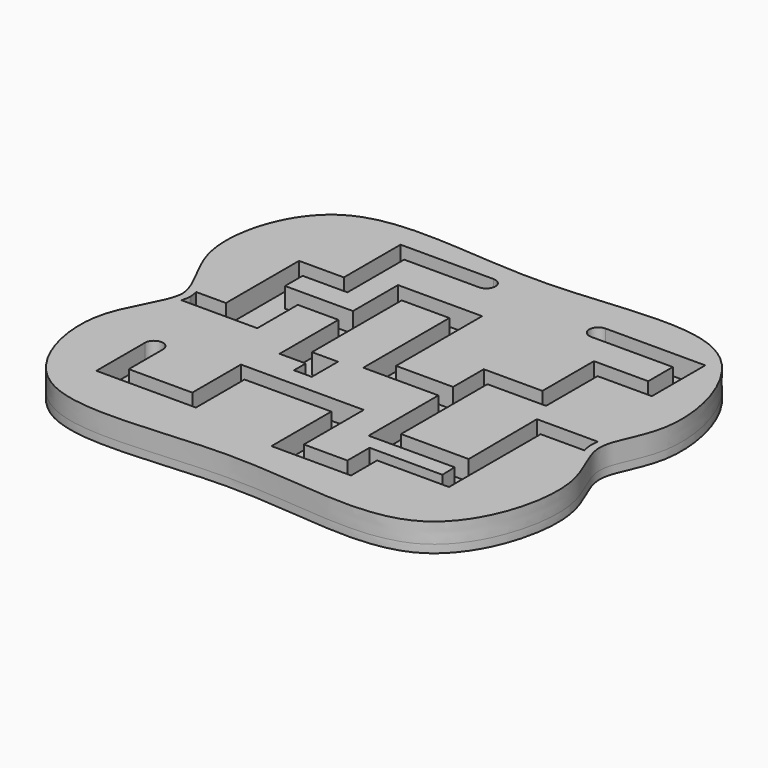
from build123d import *

# Parameters (mm, degrees)
F1_DEPTH = 5
F3_DEPTH = 2


# Not quite as in the source:
# - ends of sketch curves that miss each other by under 0.0002 mm in the source are joined
# - the dataset's text gives a spline's control points without its knots; the knots are read off the source's solid


with BuildPart() as f1:
    # F0 (on Top) → F1 (new body)
    with BuildSketch(Plane.XY):
        with BuildLine():
            add(Edge.make_bspline(
                [(-50.9456880391, 0), (-51.503372077, 5.566100958), (-62.5146563062, 16.7687371178), (-51.6356678734, 55.8412478467), (0.1475571881, 42.8791360776), (50.2128520626, 56.7362917081), (62.2679110659, 14.7606837887), (53.2085513997, 4.423548849), (53.2085513997, 0)],
                knots=[0, 0, 0, 0, 0.1323057261, 0.2944464696, 0.5028679611, 0.7079205641, 0.8788275568, 1, 1, 1, 1], degree=3))
            add(Edge.make_bspline(
                [(-50.9456880391, 0), (-51.503372077, -5.566100958), (-62.5146563062, -16.7687371178), (-51.6356678734, -55.8412478467), (0.1475571881, -42.8791360776), (50.2128520626, -56.7362917081), (62.2679110659, -14.7606837887), (53.2085513997, -4.423548849), (53.2085513997, 0)],
                knots=[0, 0, 0, 0, 0.1323057261, 0.2944464696, 0.5028679611, 0.7079205641, 0.8788275568, 1, 1, 1, 1], degree=3))
        make_face()
        with BuildLine():
            Line((-48.9556517112, -0.199387597), (-48.9556517112, 0.199387597))
            add(Edge.make_bspline(
                [(-48.9556517112, 0.199387597), (-49.0230581408, 0.872153835), (-49.1434598402, 1.5283549669), (-49.3032455355, 2.1689208225)],
                knots=[0, 0, 0, 0, 0.0134565679, 0.0134565679, 0.0134565679, 0.0134565679], degree=3))
            add(Edge.make_bspline(
                [(-49.3032455355, 2.1689208225), (-49.3289938856, 2.2721435415), (-49.5486681117, 3.1158233145), (-50.3333765859, 5.3666022776), (-51.7083191736, 8.0724029733), (-53.1209086073, 10.7900166471), (-54.129106738, 12.8665682522), (-55.0170217752, 15.0110037787), (-55.6046051051, 16.8816712621), (-55.9522945748, 18.4420782969), (-56.2119350784, 20.0683796187), (-56.3724776346, 22.2239468518), (-56.2956181819, 24.9357462684), (-55.9484823091, 27.7099356689), (-55.3327645413, 30.4826837202), (-54.1596605839, 34.0951290577), (-52.4706173692, 37.4569548645), (-50.3055678721, 40.3373443598), (-48.7651043366, 41.8945148544), (-47.4239283107, 42.9732523053), (-46.3668717243, 43.6917267161), (-45.2431785, 44.3276277734), (-42.8583955664, 45.4469740118), (-38.7592709718, 46.5788205426), (-32.3058608948, 47.1262089229), (-25.0820855304, 46.9759496812), (-17.2930636884, 46.4412854792), (-10.4881214189, 45.9507506166), (-4.9427269682, 45.7017808464), (-1.4517359227, 45.6414313985), (1.3455768971, 45.6739189351), (4.1268429052, 45.7580649245), (7.5730162875, 45.9432190449), (11.6414290853, 46.2478539423), (16.9540360773, 46.7029916702), (23.3402489636, 47.2508675251), (30.4419879804, 47.5223937353), (36.811225819, 47.0752312205), (41.3600698997, 45.8689935004), (44.1162047486, 44.4839190145), (45.5724511014, 43.5193095702), (46.9701029127, 42.4225154001), (48.6041529452, 40.8189337724), (50.9584744577, 37.8205240312), (53.3730883469, 33.4014157471), (55.3284302579, 27.5244590296), (56.1242091362, 22.5860447114), (56.2480403548, 18.8831588665), (56.1134124796, 16.729489546), (55.8816325113, 15.1445697663), (55.5699441853, 13.625327009), (55.0539456622, 11.8342505962), (54.297765853, 9.8121817564), (53.4729568569, 7.8763608061), (52.6525822662, 5.983449899), (51.9178222861, 4.0821512315), (51.5184265331, 2.6556326514), (51.3750938957, 1.8579303284), (51.35575883, 1.7403489352)],
                knots=[0.0134565679, 0.0134565679, 0.0134565679, 0.0134565679, 0.015625, 0.03125, 0.0625, 0.078125, 0.09375, 0.109375, 0.125, 0.1328125, 0.140625, 0.15625, 0.171875, 0.1875, 0.203125, 0.21875, 0.25, 0.265625, 0.28125, 0.2890625, 0.296875, 0.3046875, 0.3125, 0.34375, 0.375, 0.40625, 0.4375, 0.46875, 0.484375, 0.5, 0.5078125, 0.515625, 0.53125, 0.546875, 0.5625, 0.59375, 0.625, 0.65625, 0.6875, 0.703125, 0.7109375, 0.71875, 0.734375, 0.75, 0.78125, 0.8125, 0.84375, 0.859375, 0.875, 0.8828125, 0.890625, 0.90625, 0.921875, 0.9375, 0.953125, 0.96875, 0.984375, 0.9870602893, 0.9870602893, 0.9870602893, 0.9870602893], degree=3))
            add(Edge.make_bspline(
                [(51.35575883, 1.7403489352), (51.2698747401, 1.2180662045), (51.2172428231, 0.684051253), (51.2095357831, 0.1389744246)],
                knots=[0.9870602893, 0.9870602893, 0.9870602893, 0.9870602893, 0.9989880287, 0.9989880287, 0.9989880287, 0.9989880287], degree=3))
            Line((51.2095357831, 0.1389744246), (51.2085513997, 0))
            add(Edge.make_bspline(
                [(51.5661417074, -2.7596510648), (51.511731272, -2.5389008313), (51.3135124198, -1.6457876627), (51.2085513997, -0.7164876933), (51.2085513997, 0)],
                knots=[0.9791854168, 0.9791854168, 0.9791854168, 0.9791854168, 0.984375, 1, 1, 1, 1], degree=3))
            add(Edge.make_bspline(
                [(-49.3446149503, -2.3310785091), (-49.3573549812, -2.3799350681), (-49.566873924, -3.1680430377), (-50.3333765859, -5.3666022776), (-51.7083191736, -8.0724029733), (-53.1209086073, -10.7900166471), (-54.129106738, -12.8665682522), (-55.0170217752, -15.0110037787), (-55.6046051051, -16.8816712621), (-55.9522945748, -18.4420782969), (-56.2119350784, -20.0683796187), (-56.3724776346, -22.2239468518), (-56.2956181819, -24.9357462684), (-55.9484823091, -27.7099356689), (-55.3327645413, -30.4826837202), (-54.1596605839, -34.0951290577), (-52.4706173692, -37.4569548645), (-50.3055678721, -40.3373443598), (-48.7651043366, -41.8945148544), (-47.4239283107, -42.9732523053), (-46.3668717243, -43.6917267161), (-45.2431785, -44.3276277734), (-42.8583955664, -45.4469740118), (-38.7592709718, -46.5788205426), (-32.3058608948, -47.1262089229), (-25.0820855304, -46.9759496812), (-17.2930636884, -46.4412854792), (-10.4881214189, -45.9507506166), (-4.9427269682, -45.7017808464), (-1.4517359227, -45.6414313985), (1.3455768971, -45.6739189351), (4.1268429052, -45.7580649245), (7.5730162875, -45.9432190449), (11.6414290853, -46.2478539423), (16.9540360773, -46.7029916702), (23.3402489636, -47.2508675251), (30.4419879804, -47.5223937353), (36.811225819, -47.0752312205), (41.3600698997, -45.8689935004), (44.1162047486, -44.4839190145), (45.5724511014, -43.5193095702), (46.9701029127, -42.4225154001), (48.6041529452, -40.8189337724), (50.9584744577, -37.8205240312), (53.3730883469, -33.4014157471), (55.3284302579, -27.5244590296), (56.1242091362, -22.5860447114), (56.2480403548, -18.8831588665), (56.1134124796, -16.729489546), (55.8816325113, -15.1445697663), (55.5699441853, -13.625327009), (55.0539456622, -11.8342505962), (54.297765853, -9.8121817564), (53.4729568569, -7.8763608061), (52.6525822662, -5.983449899), (51.9991683774, -4.292646113), (51.6755523391, -3.2035442686), (51.5661417074, -2.7596510648)],
                knots=[0.0145944116, 0.0145944116, 0.0145944116, 0.0145944116, 0.015625, 0.03125, 0.0625, 0.078125, 0.09375, 0.109375, 0.125, 0.1328125, 0.140625, 0.15625, 0.171875, 0.1875, 0.203125, 0.21875, 0.25, 0.265625, 0.28125, 0.2890625, 0.296875, 0.3046875, 0.3125, 0.34375, 0.375, 0.40625, 0.4375, 0.46875, 0.484375, 0.5, 0.5078125, 0.515625, 0.53125, 0.546875, 0.5625, 0.59375, 0.625, 0.65625, 0.6875, 0.703125, 0.7109375, 0.71875, 0.734375, 0.75, 0.78125, 0.8125, 0.84375, 0.859375, 0.875, 0.8828125, 0.890625, 0.90625, 0.921875, 0.9375, 0.953125, 0.96875, 0.9791854168, 0.9791854168, 0.9791854168, 0.9791854168], degree=3))
            add(Edge.make_bspline(
                [(-48.9556517112, -0.199387597), (-49.0287578091, -0.9290407592), (-49.1642003, -1.6392089944), (-49.3446149503, -2.3310785091)],
                knots=[0, 0, 0, 0, 0.0145944116, 0.0145944116, 0.0145944116, 0.0145944116], degree=3))
        make_face(mode=Mode.SUBTRACT)
        with BuildLine():
            Line((-13.7496860698, -11.7393117398), (-13.7558765718, -11.7393396612))
            Line((-13.7558765718, -11.7393396612), (-23.7765221646, -11.784536536))
            Line((-23.7765221646, -11.784536536), (-23.7765440643, -4.1925245896))
            Line((-23.7765440643, -4.1925245896), (-45.4828031361, -4.1925245896))
            ThreePointArc((-45.4828031361, -4.1925245896), (-47.7328031361, -6.4425245896), (-45.4828031361, -8.6925245896))
            Line((-45.4828031361, -8.6925245896), (-28.2765440643, -8.6925245896))
            Line((-28.2765440643, -8.6925245896), (-28.2765440643, -16.3048788162))
            Line((-28.2765440643, -16.3048788162), (-23.3427176327, -16.2988154143))
            Line((-23.3427176327, -16.2988154143), (7.32941553, -16.2988154143))
            Line((7.32941553, -16.2988154143), (7.32941553, -34.9776947796))
            Line((7.32941553, -34.9776947796), (18.1962005645, -34.9776947796))
            Line((18.1962005645, -34.9776947796), (18.1962005645, -28.0615705997))
            Line((18.1962005645, -28.0615705997), (36.4300050671, -28.1137742644))
            Line((36.4300050671, -28.1137742644), (36.3082401454, -24.1376161575))
            Line((36.3082401454, -24.1376161575), (14.8714620192, -24.2085577739))
            Line((14.8714620192, -24.2085577739), (14.8714620192, -2.4310778646))
            Line((14.8714620192, -2.4310778646), (-3.8760740971, -2.4310778646))
            Line((-3.8760740971, -2.4310778646), (-3.8760740971, 24.4457749831))
            Line((-3.8760740971, 24.4457749831), (-15.7917661872, 24.4457749831))
            Line((-15.7917661872, 24.4457749831), (-15.7917661872, 10.4851193981))
            Line((-15.7917661872, 10.4851193981), (-15.7917661872, -3.5465050414))
            Line((-15.7917661872, -3.5465050414), (-9.3074124306, -3.5465050414))
            Line((-9.3074124306, -3.5465050414), (-9.3074124306, -11.7159346119))
            Line((-9.3074124306, -11.7159346119), (-13.7496860698, -11.7393117398))
        make_face()
        with BuildLine():
            Line((-30.4350983351, -2.3310791776), (-49.3446149503, -2.3310791776))
            add(Edge.make_bspline(
                [(-49.3446149503, -2.3310791776), (-49.3573549812, -2.3799350681), (-49.566873924, -3.1680430377), (-50.3333765859, -5.3666022776), (-51.7083191736, -8.0724029733), (-53.1209086073, -10.7900166471), (-54.129106738, -12.8665682522), (-55.0170217752, -15.0110037787), (-55.6046051051, -16.8816712621), (-55.9522945748, -18.4420782969), (-56.2119350784, -20.0683796187), (-56.3724776346, -22.2239468518), (-56.2956181819, -24.9357462684), (-55.9484823091, -27.7099356689), (-55.3327645413, -30.4826837202), (-54.1596605839, -34.0951290577), (-52.4706173692, -37.4569548645), (-50.3055678721, -40.3373443598), (-48.7651043366, -41.8945148544), (-47.4239283107, -42.9732523053), (-46.3668717243, -43.6917267161), (-45.2431785, -44.3276277734), (-42.8583955664, -45.4469740118), (-38.7592709718, -46.5788205426), (-32.3058608948, -47.1262089229), (-25.0820855304, -46.9759496812), (-17.2930636884, -46.4412854792), (-10.4881214189, -45.9507506166), (-4.9427269682, -45.7017808464), (-1.4517359227, -45.6414313985), (1.3455768971, -45.6739189351), (4.1268429052, -45.7580649245), (7.5730162875, -45.9432190449), (11.6414290853, -46.2478539423), (16.9540360773, -46.7029916702), (23.3402489636, -47.2508675251), (30.4419879804, -47.5223937353), (36.811225819, -47.0752312205), (41.3600698997, -45.8689935004), (44.1162047486, -44.4839190145), (45.5724511014, -43.5193095702), (46.9701029127, -42.4225154001), (48.6041529452, -40.8189337724), (50.9584744577, -37.8205240312), (53.3730883469, -33.4014157471), (55.3284302579, -27.5244590296), (56.1242091362, -22.5860447114), (56.2480403548, -18.8831588665), (56.1134124796, -16.729489546), (55.8816325113, -15.1445697663), (55.5699441853, -13.625327009), (55.0539456622, -11.8342505962), (54.297765853, -9.8121817564), (53.4729568569, -7.8763608061), (52.6525822662, -5.983449899), (51.9991683774, -4.292646113), (51.6755523391, -3.2035442686), (51.5661417074, -2.7596510648)],
                knots=[0.0145944116, 0.0145944116, 0.0145944116, 0.0145944116, 0.015625, 0.03125, 0.0625, 0.078125, 0.09375, 0.109375, 0.125, 0.1328125, 0.140625, 0.15625, 0.171875, 0.1875, 0.203125, 0.21875, 0.25, 0.265625, 0.28125, 0.2890625, 0.296875, 0.3046875, 0.3125, 0.34375, 0.375, 0.40625, 0.4375, 0.46875, 0.484375, 0.5, 0.5078125, 0.515625, 0.53125, 0.546875, 0.5625, 0.59375, 0.625, 0.65625, 0.6875, 0.703125, 0.7109375, 0.71875, 0.734375, 0.75, 0.78125, 0.8125, 0.84375, 0.859375, 0.875, 0.8828125, 0.890625, 0.90625, 0.921875, 0.9375, 0.953125, 0.96875, 0.9791854168, 0.9791854168, 0.9791854168, 0.9791854168], degree=3))
            Line((51.5661417074, -2.7596510648), (40.6783057892, -2.7596510648))
            Line((40.6783057892, -2.7596510648), (40.6508542392, -31.3410854042))
            Line((40.6508542392, -31.3410854042), (22.6962005645, -31.3410854042))
            Line((22.6962005645, -31.3410854042), (22.6962005645, -39.4776947796))
            Line((22.6962005645, -39.4776947796), (2.82941553, -39.4776947796))
            Line((2.82941553, -39.4776947796), (2.82941553, -20.7988154143))
            Line((2.82941553, -20.7988154143), (-18.8427176327, -20.7988154143))
            Line((-18.8427176327, -20.7988154143), (-18.8427176327, -35.9753966331))
            Line((-18.8427176327, -35.9753966331), (-43.7046626657, -35.9753966331))
            Line((-43.7046626657, -35.9753966331), (-43.7046626657, -20.7988154143))
            ThreePointArc((-43.7046626657, -20.7988154143), (-41.4546626657, -18.5488154143), (-39.2046626657, -20.7988154143))
            Line((-39.2046626657, -20.7988154143), (-39.2046626657, -31.4753966331))
            Line((-39.2046626657, -31.4753966331), (-23.3427176327, -31.4753966331))
            Line((-23.3427176327, -31.4753966331), (-23.3427176327, -16.2988154143))
            Line((-23.3427176327, -16.2988154143), (-28.2765440643, -16.3048788162))
            Line((-28.2765440643, -16.3048788162), (-28.2765440643, -8.6925245896))
            Line((-28.2765440643, -8.6925245896), (-45.4828031361, -8.6925245896))
            ThreePointArc((-45.4828031361, -8.6925245896), (-47.7328031361, -6.4425245896), (-45.4828031361, -4.1925245896))
            Line((-45.4828031361, -4.1925245896), (-23.7765440643, -4.1925245896))
            Line((-23.7765440643, -4.1925245896), (-23.7765440643, -11.784536441))
            Line((-23.7765440643, -11.784536441), (-13.7558765709, -11.7393398549))
            Line((-13.7558765709, -11.7393398549), (-13.7558765709, -8.0465046149))
            Line((-13.7558765709, -8.0465046149), (-20.2917661872, -8.0465050414))
            Line((-20.2917661872, -8.0465050414), (-20.2917661872, 10.3210946521))
            Line((-20.2917661872, 10.3210946521), (-30.4350983351, 10.3210946521))
            Line((-30.4350983351, 10.3210946521), (-30.4350983351, -2.3310791776))
        make_face()
        with BuildLine():
            add(Edge.make_bspline(
                [(-49.3032455355, 2.1689208225), (-49.3289938856, 2.2721435415), (-49.5486681117, 3.1158233145), (-50.3333765859, 5.3666022776), (-51.7083191736, 8.0724029733), (-53.1209086073, 10.7900166471), (-54.129106738, 12.8665682522), (-55.0170217752, 15.0110037787), (-55.6046051051, 16.8816712621), (-55.9522945748, 18.4420782969), (-56.2119350784, 20.0683796187), (-56.3724776346, 22.2239468518), (-56.2956181819, 24.9357462684), (-55.9484823091, 27.7099356689), (-55.3327645413, 30.4826837202), (-54.1596605839, 34.0951290577), (-52.4706173692, 37.4569548645), (-50.3055678721, 40.3373443598), (-48.7651043366, 41.8945148544), (-47.4239283107, 42.9732523053), (-46.3668717243, 43.6917267161), (-45.2431785, 44.3276277734), (-42.8583955664, 45.4469740118), (-38.7592709718, 46.5788205426), (-32.3058608948, 47.1262089229), (-25.0820855304, 46.9759496812), (-17.2930636884, 46.4412854792), (-10.4881214189, 45.9507506166), (-4.9427269682, 45.7017808464), (-1.4517359227, 45.6414313985), (1.3455768971, 45.6739189351), (4.1268429052, 45.7580649245), (7.5730162875, 45.9432190449), (11.6414290853, 46.2478539423), (16.9540360773, 46.7029916702), (23.3402489636, 47.2508675251), (30.4419879804, 47.5223937353), (36.811225819, 47.0752312205), (41.3600698997, 45.8689935004), (44.1162047486, 44.4839190145), (45.5724511014, 43.5193095702), (46.9701029127, 42.4225154001), (48.6041529452, 40.8189337724), (50.9584744577, 37.8205240312), (53.3730883469, 33.4014157471), (55.3284302579, 27.5244590296), (56.1242091362, 22.5860447114), (56.2480403548, 18.8831588665), (56.1134124796, 16.729489546), (55.8816325113, 15.1445697663), (55.5699441853, 13.625327009), (55.0539456622, 11.8342505962), (54.297765853, 9.8121817564), (53.4729568569, 7.8763608061), (52.6525822662, 5.983449899), (51.9178222861, 4.0821512315), (51.5184265331, 2.6556326514), (51.3750938957, 1.8579303284), (51.35575883, 1.7403489352)],
                knots=[0.0134565679, 0.0134565679, 0.0134565679, 0.0134565679, 0.015625, 0.03125, 0.0625, 0.078125, 0.09375, 0.109375, 0.125, 0.1328125, 0.140625, 0.15625, 0.171875, 0.1875, 0.203125, 0.21875, 0.25, 0.265625, 0.28125, 0.2890625, 0.296875, 0.3046875, 0.3125, 0.34375, 0.375, 0.40625, 0.4375, 0.46875, 0.484375, 0.5, 0.5078125, 0.515625, 0.53125, 0.546875, 0.5625, 0.59375, 0.625, 0.65625, 0.6875, 0.703125, 0.7109375, 0.71875, 0.734375, 0.75, 0.78125, 0.8125, 0.84375, 0.859375, 0.875, 0.8828125, 0.890625, 0.90625, 0.921875, 0.9375, 0.953125, 0.96875, 0.984375, 0.9870602893, 0.9870602893, 0.9870602893, 0.9870602893], degree=3))
            Line((-49.3032455355, 2.1689208225), (-41.857537305, 2.1689221593))
            Line((-41.857537305, 2.1689221593), (-41.857537305, 14.9851193981))
            Line((-41.857537305, 14.9851193981), (-41.857537305, 24.9801719891))
            Line((-41.857537305, 24.9801719891), (-30.6648744699, 24.9801719891))
            Line((-30.6648744699, 24.9801719891), (-30.6648744699, 42.686752975))
            Line((-30.6648744699, 42.686752975), (-7.4470443651, 42.686752975))
            ThreePointArc((-7.4470443651, 42.686752975), (-5.1970435306, 40.4367521405), (-7.4470443651, 38.1867513061))
            Line((-7.4470443651, 38.1867513061), (-26.1648744699, 38.1867513061))
            Line((-26.1648744699, 38.1867513061), (-26.1648744699, 20.4801719891))
            Line((-26.1648744699, 20.4801719891), (-37.357537305, 20.4801719891))
            Line((-37.357537305, 20.4801719891), (-37.357537305, 14.9851193981))
            Line((-37.357537305, 14.9851193981), (-20.391766211, 14.9851193981))
            Line((-20.391766211, 14.9851193981), (-20.391766211, 29.0457750069))
            Line((-20.391766211, 29.0457750069), (0.6239259029, 29.0457750069))
            Line((0.6239259029, 29.0457750069), (0.6239259029, 28.9457749831))
            Line((0.6239259029, 28.9457749831), (0.6239259029, 2.1689221593))
            Line((0.6239259029, 2.1689221593), (14.8714622483, 2.1689221593))
            Line((14.8714622483, 2.1689221593), (14.8714622483, 11.7463534698))
            Line((14.8714622483, 11.7463534698), (29.520897001, 11.7463527322))
            Line((29.520897001, 11.7463527322), (29.520897001, 27.8253797442))
            Line((29.520897001, 27.8253797442), (43.0820547044, 27.8253797442))
            Line((43.0820547044, 27.8253797442), (43.0820547044, 35.5007573962))
            Line((43.0820547044, 35.5007573962), (22.6809028536, 35.5007573962))
            ThreePointArc((22.6809028536, 35.5007573962), (20.4309028536, 37.7507573962), (22.6809028536, 40.0007573962))
            Line((22.6809028536, 40.0007573962), (47.5820547044, 40.0007573962))
            Line((47.5820547044, 40.0007573962), (47.5820547044, 23.3253797442))
            Line((47.5820547044, 23.3253797442), (34.020897001, 23.3253797442))
            Line((34.020897001, 23.3253797442), (34.020897001, 7.2463527322))
            Line((34.020897001, 7.2463527322), (19.3714620192, 7.2463527322))
            Line((19.3714620192, 7.2463527322), (19.3714620192, 2.1689221593))
            Line((19.3714620192, 2.1689221593), (19.3714620192, -19.5085577263))
            Line((19.3714620192, -19.5085577263), (19.3714620192, -19.7085577739))
            Line((19.3714620192, -19.7085577739), (36.2813561411, -19.7172500466))
            Line((36.2813561411, -19.7172500466), (36.1508542392, 1.7403489352))
            Line((36.1508542392, 1.7403489352), (51.35575883, 1.7403489352))
        make_face()
    extrude(amount=F1_DEPTH)

    # F2 (on Top) → F3 (join)
    with BuildSketch(Plane.XY):
        with BuildLine():
            add(Edge.make_bspline(
                [(-50.9456880391, 0), (-51.503372077, 5.566100958), (-62.5146563062, 16.7687371178), (-51.6356678734, 55.8412478467), (0.1475571881, 42.8791360776), (50.2128520626, 56.7362917081), (62.2679110659, 14.7606837887), (53.2085513997, 4.423548849), (53.2085513997, 0)],
                knots=[0, 0, 0, 0, 0.1323057261, 0.2944464696, 0.5028679611, 0.7079205641, 0.8788275568, 1, 1, 1, 1], degree=3))
            add(Edge.make_bspline(
                [(-50.9456880391, 0), (-51.503372077, -5.566100958), (-62.5146563062, -16.7687371178), (-51.6356678734, -55.8412478467), (0.1475571881, -42.8791360776), (50.2128520626, -56.7362917081), (62.2679110659, -14.7606837887), (53.2085513997, -4.423548849), (53.2085513997, 0)],
                knots=[0, 0, 0, 0, 0.1323057261, 0.2944464696, 0.5028679611, 0.7079205641, 0.8788275568, 1, 1, 1, 1], degree=3))
        make_face()
    extrude(amount=-F3_DEPTH)


solid = f1.part
